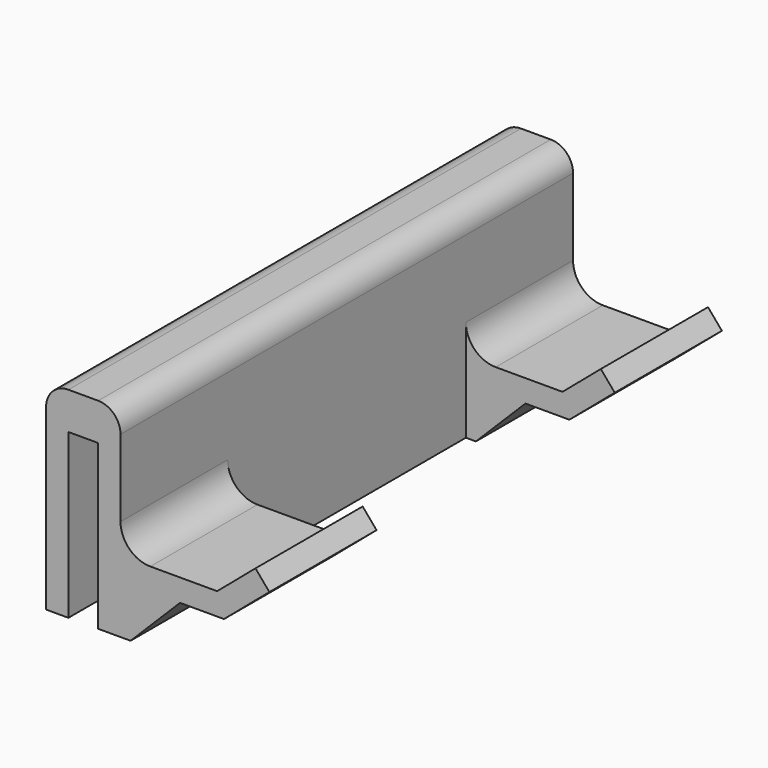
from build123d import *

# Parameters (mm, degrees)
F1_DEPTH    = 38
F3_DEPTH    = 50
F4_T4_DEPTH = 9
F4_T9_DEPTH = 9
F5_W        = 38
F5_H        = 14.5097850376
F6_DEPTH    = 25
F7_R        = 2
F8_R        = 1.5


# Not quite as in the source:
# - a fillet or chamfer that OpenCascade refuses, or shapes differently, is made with other operations: its cross-section is extruded or revolved along the edge and cut away or added


with BuildPart() as f1:
    # F0 (on Front) → F1 (new body)
    with BuildSketch(Plane.XZ):
        Polygon((0, 16.9122221599), (0, -11.0877778401), (1.5, -11.0877778401), (1.5, 14.4122221599), (3.5, 14.4122221599), (3.5, 3.4220071975), (5, 3.4220071975), (5, 6.7475574595), (5, 8.2475574595), (5, 16.9122221599), align=None)
        Polygon((11.4920105912, 8.2475574595), (5, 8.2475574595), (5, 6.7475574595), (11.9522421048, 6.7475574595), (15, 9.3381504056), (14.0667535676, 10.4360879209), align=None)
    extrude(amount=F1_DEPTH)

    # F2 (on face) → F3 (cut)
    with BuildSketch(Plane.XY.offset(16.9122221599)):
        Polygon((16.5792163461, -29), (16.5792163461, -19), (16.5792163461, -9), (5, -9), (5, -29), align=None)
    extrude(amount=-F3_DEPTH, mode=Mode.SUBTRACT)

    # F4: chamfer of 4 on 2 edges, made by hand


with BuildPart() as f4_tool2:
    # F4_s3 → F4_t4 (new body)
    with BuildSketch(Plane.XZ.offset(29)):
        Polygon((9, 6.7475574595), (5, 2.7475574595), (5, 6.7475574595), align=None)
    extrude(amount=F4_T4_DEPTH)

    split(bisect_by=Plane.XY.offset(3.4220071975), keep=Keep.TOP)


with BuildPart() as f1_1:
    add(f1.part)

    # F4_t1: union F4_tool2
    add(f4_tool2.part)


with BuildPart() as f4_tool7:
    # F4_s8 → F4_t9 (new body)
    with BuildSketch(Plane.XZ):
        Polygon((5, 2.7475574595), (9, 6.7475574595), (5, 6.7475574595), align=None)
    extrude(amount=F4_T9_DEPTH)

    split(bisect_by=Plane.XY.offset(3.4220071975), keep=Keep.TOP)


with BuildPart() as f1_2:
    add(f1_1.part)

    # F4_t6: union F4_tool7
    add(f4_tool7.part)

    # F5 (on face) → F6 (cut)
    with BuildSketch(Plane.YZ.offset(1.5)):
        with Locations((-19, -3.8328853213)):
            Rectangle(F5_W, F5_H)
    extrude(amount=-F6_DEPTH, mode=Mode.SUBTRACT)

    # F7
    f7_edges = [f1_2.edges().sort_by_distance(p)[0] for p in [
        (5, -33.5, 8.247557),
        (5, -4.5, 8.247557),
    ]]
    fillet(f7_edges, radius=F7_R)

    # F8
    f8_edges = [f1_2.edges().sort_by_distance(p)[0] for p in [
        (5, -19, 16.912222),
        (0, -19, 16.912222),
    ]]
    fillet(f8_edges, radius=F8_R)


solid = f1_2.part
